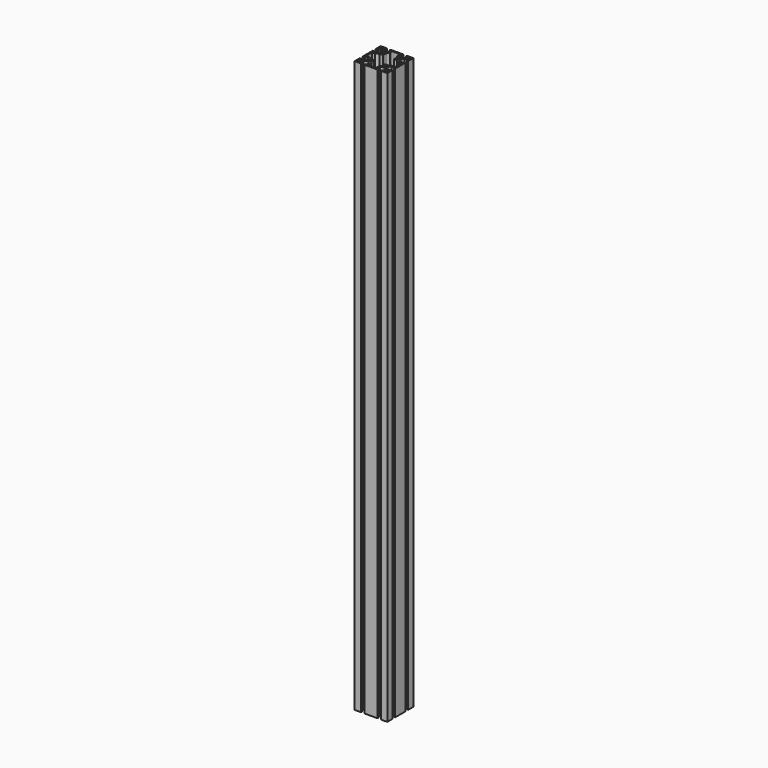
from build123d import *

# Parameters (mm, degrees)
F0_R     = 3
F0_R_2   = 2.5
F1_DEPTH = 1050
F2_R     = 2
F3_R     = 7


# Not quite as in the source:
# - a feature names something its author has since deleted; it is built from what else it names


with BuildPart() as f1:
    # F0 (on Top) → F1 (new body)
    with BuildSketch(Plane.XY):
        with BuildLine():
            Line((18.15, -30), (30, -30))
            Line((30, -30), (30, -18.15))
            Line((30, -18.15), (27.5, -18.15))
            Line((27.5, -18.15), (27.5, -20.15))
            Line((27.5, -20.15), (21.5477069044, -20.15))
            ThreePointArc((21.5477069044, -20.15), (19.5, -15), (21.5477069044, -9.85))
            Line((21.5477069044, -9.85), (27.5, -9.85))
            Line((27.5, -9.85), (27.5, -11.85))
            Line((27.5, -11.85), (30, -11.85))
            Line((30, -11.85), (30, 11.85))
            Line((30, 11.85), (27.5, 11.85))
            Line((27.5, 11.85), (27.5, 9.85))
            Line((27.5, 9.85), (21.5477069044, 9.85))
            ThreePointArc((21.5477069044, 9.85), (19.5, 15), (21.5477069044, 20.15))
            Line((21.5477069044, 20.15), (27.5, 20.15))
            Line((27.5, 20.15), (27.5, 18.15))
            Line((27.5, 18.15), (30, 18.15))
            Line((30, 18.15), (30, 30))
            Line((30, 30), (18.15, 30))
            Line((18.15, 30), (18.15, 27.5))
            Line((18.15, 27.5), (20.15, 27.5))
            Line((20.15, 27.5), (20.15, 21.5477069044))
            ThreePointArc((20.15, 21.5477069044), (15, 19.5), (9.85, 21.5477069044))
            Line((9.85, 21.5477069044), (9.85, 27.5))
            Line((9.85, 27.5), (11.85, 27.5))
            Line((11.85, 27.5), (11.85, 30))
            Line((11.85, 30), (-11.85, 30))
            Line((-11.85, 30), (-11.85, 27.5))
            Line((-11.85, 27.5), (-9.85, 27.5))
            Line((-9.85, 27.5), (-9.85, 21.5477069044))
            ThreePointArc((-9.85, 21.5477069044), (-15, 19.5), (-20.15, 21.5477069044))
            Line((-20.15, 21.5477069044), (-20.15, 27.5))
            Line((-20.15, 27.5), (-18.15, 27.5))
            Line((-18.15, 27.5), (-18.15, 30))
            Line((-18.15, 30), (-30, 30))
            Line((-30, 30), (-30, 18.15))
            Line((-30, 18.15), (-27.5, 18.15))
            Line((-27.5, 18.15), (-27.5, 20.15))
            Line((-27.5, 20.15), (-21.5477069044, 20.15))
            ThreePointArc((-21.5477069044, 20.15), (-19.5, 15), (-21.5477069044, 9.85))
            Line((-21.5477069044, 9.85), (-27.5, 9.85))
            Line((-27.5, 9.85), (-27.5, 11.85))
            Line((-27.5, 11.85), (-30, 11.85))
            Line((-30, 11.85), (-30, -11.85))
            Line((-30, -11.85), (-27.5, -11.85))
            Line((-27.5, -11.85), (-27.5, -9.85))
            Line((-27.5, -9.85), (-21.5477069044, -9.85))
            ThreePointArc((-21.5477069044, -9.85), (-19.5, -15), (-21.5477069044, -20.15))
            Line((-21.5477069044, -20.15), (-27.5, -20.15))
            Line((-27.5, -20.15), (-27.5, -18.15))
            Line((-27.5, -18.15), (-30, -18.15))
            Line((-30, -18.15), (-30, -30))
            Line((-30, -30), (-18.15, -30))
            Line((-18.15, -30), (-18.15, -27.5))
            Line((-18.15, -27.5), (-20.15, -27.5))
            Line((-20.15, -27.5), (-20.15, -21.5477069044))
            ThreePointArc((-20.15, -21.5477069044), (-15, -19.5), (-9.85, -21.5477069044))
            Line((-9.85, -21.5477069044), (-9.85, -27.5))
            Line((-9.85, -27.5), (-11.85, -27.5))
            Line((-11.85, -27.5), (-11.85, -30))
            Line((-11.85, -30), (11.85, -30))
            Line((11.85, -30), (11.85, -27.5))
            Line((11.85, -27.5), (9.85, -27.5))
            Line((9.85, -27.5), (9.85, -21.5477069044))
            ThreePointArc((9.85, -21.5477069044), (15, -19.5), (20.15, -21.5477069044))
            Line((20.15, -21.5477069044), (20.15, -27.5))
            Line((20.15, -27.5), (18.15, -27.5))
            Line((18.15, -27.5), (18.15, -30))
        make_face()
        with Locations((-25, -25)):
            Circle(F0_R, mode=Mode.SUBTRACT)
        with Locations((-15, -15)):
            Circle(F0_R_2, mode=Mode.SUBTRACT)
        with Locations((25, -25)):
            Circle(F0_R, mode=Mode.SUBTRACT)
        with Locations((15, -15)):
            Circle(F0_R_2, mode=Mode.SUBTRACT)
        with Locations((-25, 25)):
            Circle(F0_R, mode=Mode.SUBTRACT)
        with Locations((-15, 15)):
            Circle(F0_R_2, mode=Mode.SUBTRACT)
        Polygon((-7, 22), (-7, 27.5), (0, 27.5), (7, 27.5), (7, 22), (10, 16), (10, 10), (16, 10), (22, 7), (27.5, 7), (27.5, 0), (27.5, -7), (22, -7), (16, -10), (10, -10), (10, -16), (7, -22), (7, -27.5), (0, -27.5), (-7, -27.5), (-7, -22), (-10, -16), (-10, -10), (-16, -10), (-22, -7), (-27.5, -7), (-27.5, 0), (-27.5, 7), (-22, 7), (-16, 10), (-10, 10), (-10, 16), align=None, mode=Mode.SUBTRACT)
        with Locations((15, 15)):
            Circle(F0_R_2, mode=Mode.SUBTRACT)
        with Locations((25, 25)):
            Circle(F0_R, mode=Mode.SUBTRACT)
    extrude(amount=F1_DEPTH)

    # F2
    f2_edges = [f1.edges().sort_by_distance(p)[0] for p in [
        (-7, 27.5, 525),
        (7, 27.5, 525),
    ]]
    fillet(f2_edges, radius=F2_R)

    # F3
    f3_edges = [f1.edges().sort_by_distance(p)[0] for p in [
        (-10, 16, 525),
        (10, 16, 525),
    ]]
    fillet(f3_edges, radius=F3_R)


solid = f1.part
